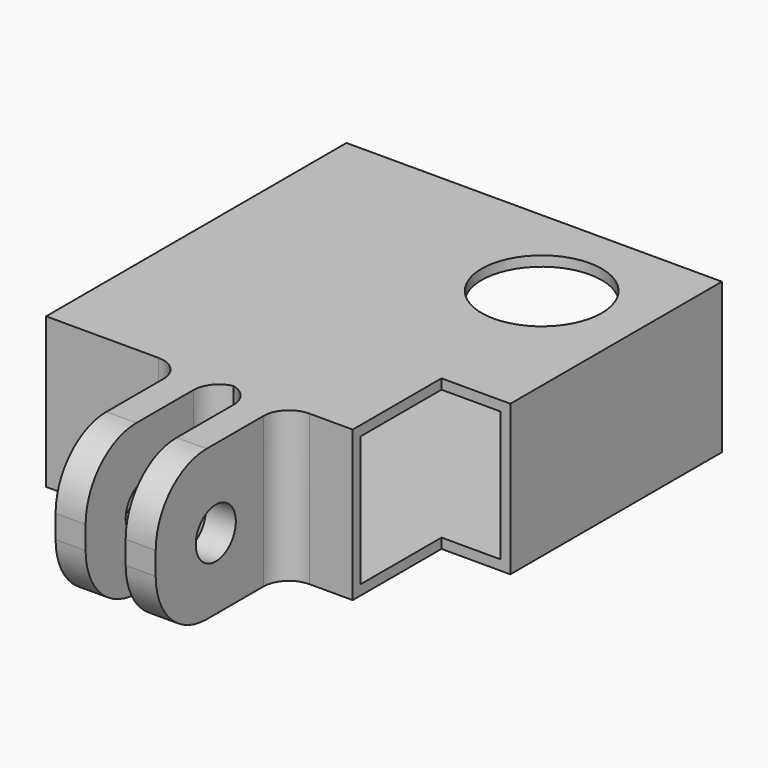
from build123d import *

# Parameters (mm, degrees)
F0_W         = 37.5
F0_H         = 37.5
F1_DEPTH     = 15
F2_W         = 35.5
F2_H         = 13
F3_DEPTH     = 36.5
F4_R         = 6
F5_DEPTH     = 1
F6_W         = 10
F6_H         = 15
F7_DEPTH     = 16
F8_R         = 2.5
F9_DEPTH     = 25.4
F10_W        = 4
F10_H        = 15
F11_DEPTH    = 16
F12_R        = 6.35
F13_W        = 6.875
F13_H        = 11.0862404108
F14_DEPTH    = 25.4
F15_T1_DEPTH = 15


# Not quite as in the source:
# - a fillet or chamfer that OpenCascade refuses, or shapes differently, is made with other operations: its cross-section is extruded or revolved along the edge and cut away or added


with BuildPart() as f1:
    # F0 (on Top) → F1 (new body)
    with BuildSketch(Plane.XY):
        with Locations((18.75, 18.75)):
            Rectangle(F0_W, F0_H)
    extrude(amount=F1_DEPTH)

    # F2 (on face) → F3 (cut)
    with BuildSketch(Plane(origin=(0, 37.5, 0), x_dir=(-1, 0, 0), z_dir=(0, 1, 0))):
        with Locations((-18.75, 7.5)):
            Rectangle(F2_W, F2_H)
    extrude(amount=-F3_DEPTH, mode=Mode.SUBTRACT)

    # F4 (on face) → F5 (cut, through all)
    with BuildSketch(Plane.XY.offset(15)):
        with Locations((27.5, 27.5)):
            Circle(F4_R)
    extrude(amount=-F5_DEPTH, mode=Mode.SUBTRACT)

    # F6 (on face) → F7 (join)
    with BuildSketch(Plane.XZ):
        with Locations((18.75, 7.5)):
            Rectangle(F6_W, F6_H)
    extrude(amount=F7_DEPTH)

    # F8 (on face) → F9 (cut)
    with BuildSketch(Plane(origin=(13.75, 0, 0), x_dir=(0, -1, 0), z_dir=(-1, 0, 0))):
        with Locations((8.5, 7.125)):
            Circle(F8_R)
    extrude(amount=-F9_DEPTH, mode=Mode.SUBTRACT)

    # F10 (on face) → F11 (cut)
    with BuildSketch(Plane.XZ.offset(16)):
        with Locations((18.75, 7.5)):
            Rectangle(F10_W, F10_H)
    extrude(amount=-F11_DEPTH, mode=Mode.SUBTRACT)

    # F12
    f12_edges = [f1.edges().sort_by_distance(p)[0] for p in [
        (15.25, -16, 15),
        (22.25, -16, 15),
        (22.25, -16, 0),
        (15.25, -16, 0),
    ]]
    fillet(f12_edges, radius=F12_R)

    # F13 (on face) → F14 (cut)
    with BuildSketch(Plane.XY.offset(15)):
        with Locations((34.0625, 5.5431202054)):
            Rectangle(F13_W, F13_H)
    extrude(amount=-F14_DEPTH, mode=Mode.SUBTRACT)

    # F15: fillet of radius 2.54 on 4 edges, made by hand

    # F15_s2 → F15_t1 (join)
    with BuildSketch(Plane.XY):
        with BuildLine():
            ThreePointArc((26.29, 0), (24.4939487758, -0.7439487758), (23.75, -2.54))
            Line((23.75, -2.54), (23.75, 0))
            Line((23.75, 0), (26.29, 0))
        make_face()
        with BuildLine():
            ThreePointArc((20.75, -2.54), (20.0060512242, -0.7439487758), (18.21, 0))
            Line((18.21, 0), (20.75, 0))
            Line((20.75, 0), (20.75, -2.54))
        make_face()
        with BuildLine():
            ThreePointArc((13.75, -2.54), (13.0060512242, -0.7439487758), (11.21, 0))
            Line((11.21, 0), (13.75, 0))
            Line((13.75, 0), (13.75, -2.54))
        make_face()
        with BuildLine():
            ThreePointArc((19.29, 0), (17.4939487758, -0.7439487758), (16.75, -2.54))
            Line((16.75, -2.54), (16.75, 0))
            Line((16.75, 0), (19.29, 0))
        make_face()
    extrude(amount=F15_T1_DEPTH)


solid = f1.part
